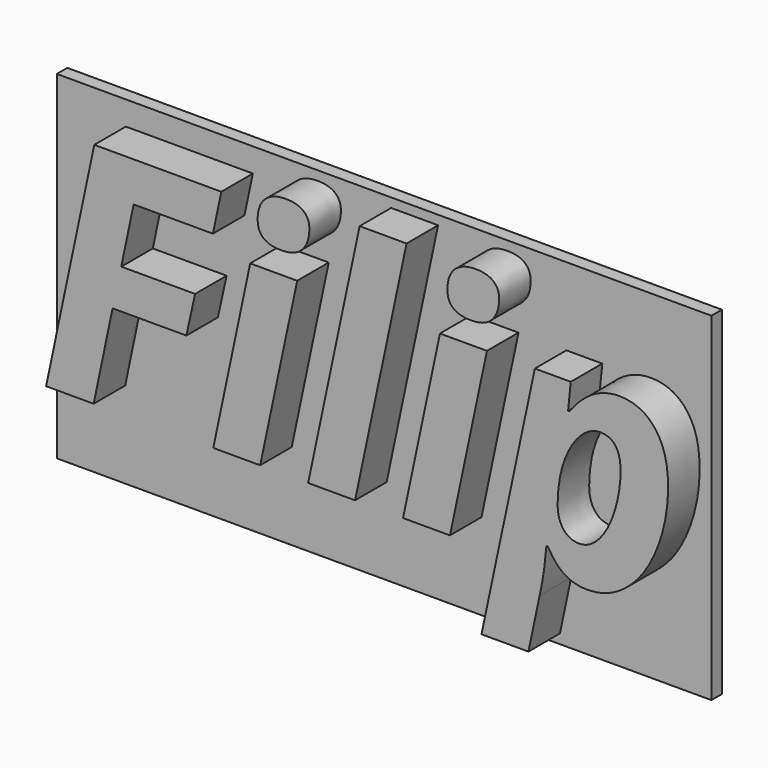
from build123d import *

# Parameters (mm, degrees)
F0_TEXT_SIZE = 24.314187174
F1_DEPTH     = 3
F2_W         = 49.7961081564
F2_H         = 25.746084284
F3_DEPTH     = 1


# Not quite as in the source:
# - Text() gives the source's letters only with a copy of the font that has no kerning and outlines rounded to 1/6400 em; it was checked with that copy


with BuildPart() as f1:
    # F0 (on Front) → F1 (new body)
    with BuildSketch(Plane.XZ):
        with Locations((-44.7518088037, -0.1232831214)):
            Text('Filip', F0_TEXT_SIZE, font='Open Sans', font_style=FontStyle.BOLDITALIC, text_align=(TextAlign.LEFT, TextAlign.BOTTOM))
    extrude(amount=F1_DEPTH)

    # F2 (on face) → F3 (join)
    with BuildSketch(Plane.XZ):
        with Locations((-20.8050888032, 6.1829204205)):
            Rectangle(F2_W, F2_H)
    extrude(amount=-F3_DEPTH)


solid = f1.part
